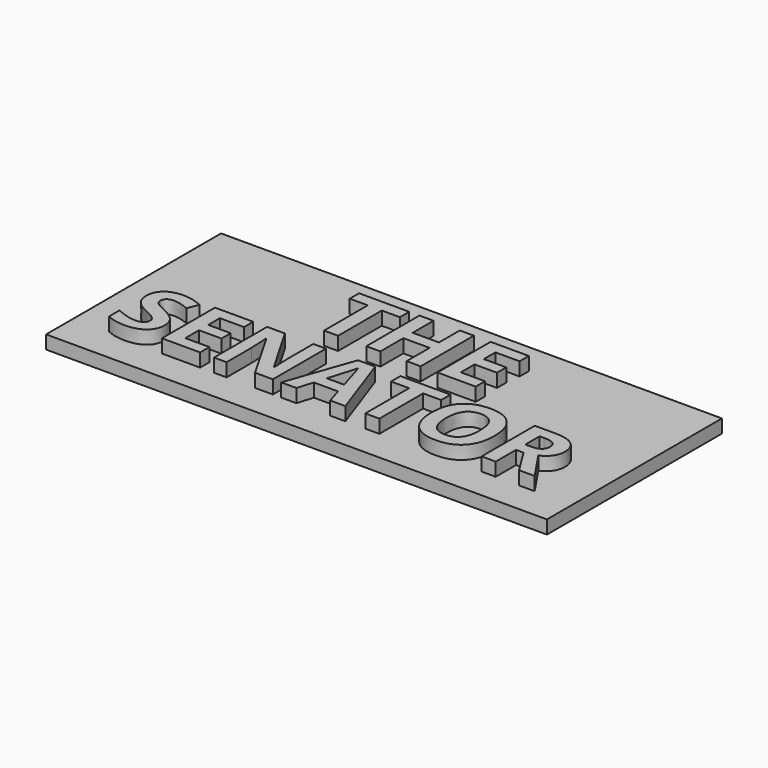
from build123d import *

# Parameters (mm, degrees)
F0_W         = 112.2
F0_H         = 49
F1_DEPTH     = 3
F2_TEXT_SIZE = 20.8333333333
F3_DEPTH     = 3


# Not quite as in the source:
# - Text() gives the source's letters only with a copy of the font that has no kerning and outlines rounded to 1/6400 em; it was checked with that copy


with BuildPart() as f1:
    # F0 (on Top) → F1 (new body)
    with BuildSketch(Plane.XY):
        Rectangle(F0_W, F0_H)
    extrude(amount=F1_DEPTH)

    # F2 (on face) → F3 (join)
    with BuildSketch(Plane.XY.offset(3)):
        with Locations((-19.8958333333, 2.5)):
            Text('THE', F2_TEXT_SIZE, font='Open Sans', font_style=FontStyle.BOLD, text_align=(TextAlign.LEFT, TextAlign.BOTTOM))
        with Locations((-49.1015625, -17.5)):
            Text('SENATOR', F2_TEXT_SIZE, font='Open Sans', font_style=FontStyle.BOLD, text_align=(TextAlign.LEFT, TextAlign.BOTTOM))
    extrude(amount=F3_DEPTH)


solid = f1.part
